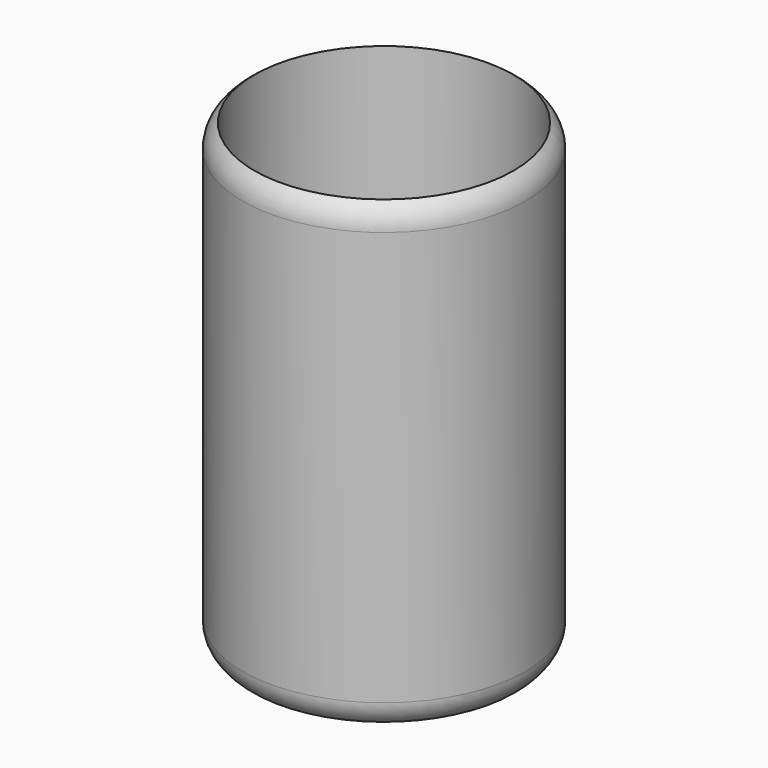
from build123d import *

# Parameters (mm, degrees)
F0_R     = 38.1
F0_R_2   = 34.925
F1_DEPTH = 123.825
F2_DEPTH = 9.525


# Not quite as in the source:
# - a fillet or chamfer that OpenCascade refuses, or shapes differently, is made with other operations: its cross-section is extruded or revolved along the edge and cut away or added


with BuildPart() as f1:
    # F0 (on Top) → F1 (new body)
    with BuildSketch(Plane.XY):
        Circle(F0_R)
        Circle(F0_R_2, mode=Mode.SUBTRACT)
    extrude(amount=F1_DEPTH)

    # F3: fillet of radius 7.62 on 1 edges, made by hand

    # F3_s1 → F3_t2 (revolve, cut)
    with BuildSketch(Plane.XZ):
        with BuildLine():
            ThreePointArc((38.1, 117.635785591), (37.25994469, 121.1138238312), (34.925, 123.825))
            Line((34.925, 123.825), (38.1, 123.825))
            Line((38.1, 123.825), (38.1, 117.635785591))
        make_face()
    revolve(axis=Axis((0, 0, 123.825), (0, 0, 1)), mode=Mode.SUBTRACT)

    # F4: fillet of radius 7.62 on 1 edges, made by hand

    # F4_s1 → F4_t2 (revolve, cut)
    with BuildSketch(Plane.XZ):
        with BuildLine():
            ThreePointArc((38.1, 6.189214409), (37.25994469, 2.7111761688), (34.925, 0))
            Line((34.925, 0), (38.1, 0))
            Line((38.1, 0), (38.1, 6.189214409))
        make_face()
    revolve(axis=Axis((0, 0, 0), (0, 0, 1)), mode=Mode.SUBTRACT)


with BuildPart() as f2:
    # F0 (on Top) → F2 (new body)
    with BuildSketch(Plane.XY):
        Circle(F0_R_2)
    extrude(amount=F2_DEPTH)


solid = Compound([f1.part, f2.part])
